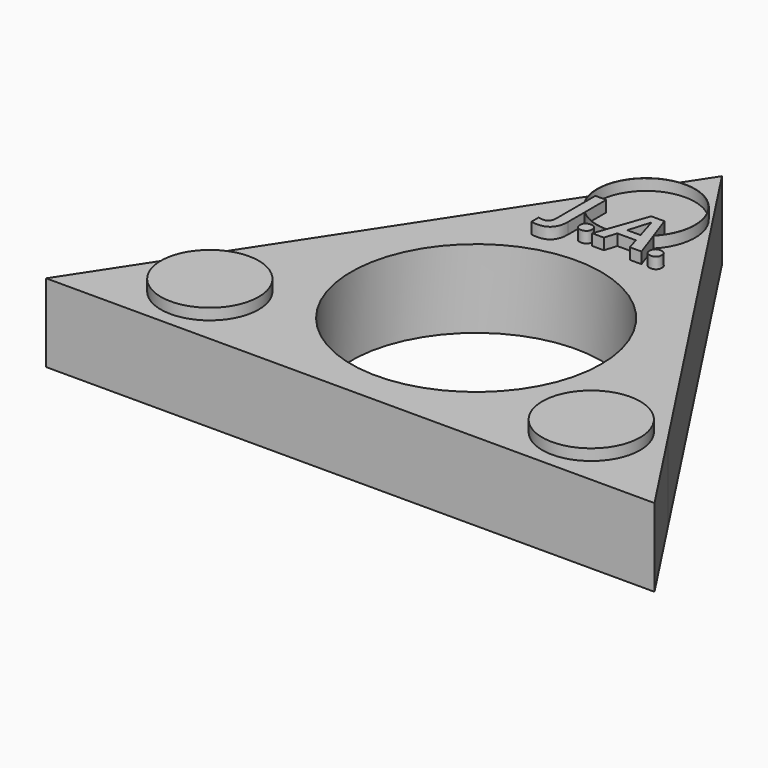
from build123d import *

# Parameters (mm, degrees)
F0_R         = 11.2
F1_DEPTH     = 7
F2_R         = 4.3842888076
F2_R_2       = 4.3652716242
F3_DEPTH     = 8
F4_TEXT_SIZE = 6.4013718252
F5_DEPTH     = 8


# Not quite as in the source:
# - the program builds the solid bodies; features that only make, move or delete a surface that nothing else refers to are left out
# - Text() gives the source's letters only with a copy of the font that has no kerning and outlines rounded to 1/6400 em; it was checked with that copy


with BuildPart() as f1:
    # F0 (on Top) → F1 (new body)
    with BuildSketch(Plane.XY):
        Polygon((21.7805314082, -5.7396855932), (0, 27.5202170014), (-27.2504271302, -14.0924753167), (27.2504271302, -14.0924753167), align=None)
        Circle(F0_R, mode=Mode.SUBTRACT)
    extrude(amount=F1_DEPTH)

    # F2 (on Top) → F3 (join)
    with BuildSketch(Plane.XY):
        with Locations((-17.0604567975, -8.4989378229)):
            Circle(F2_R)
        with Locations((-0.0203377983, 19.0601866893)):
            Circle(F2_R)
        with Locations((-0.0203377983, 19.0601866893)):
            Circle(F2_R_2, mode=Mode.SUBTRACT)
        with Locations((17.0785551781, -8.4625104598)):
            Circle(F2_R)
    extrude(amount=F3_DEPTH)

    # F4 (on Top) → F5 (join)
    with BuildSketch(Plane.XY):
        with Locations((-4.4246318284, 13.5951471457)):
            Text('J.A.', F4_TEXT_SIZE, font='Open Sans', font_style=FontStyle.BOLD, text_align=(TextAlign.LEFT, TextAlign.BOTTOM))
    extrude(amount=F5_DEPTH)


solid = f1.part
